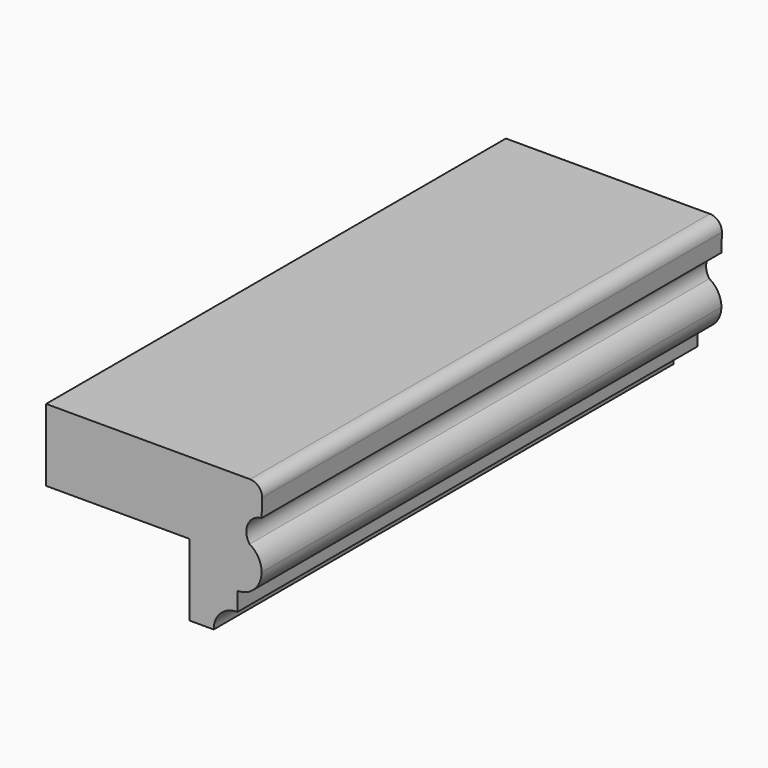
from build123d import *

# Parameters (mm, degrees)
F0_W     = 38.0493849516
F0_H     = 19.1407520324
F1_DEPTH = 152.4


# Not quite as in the source:
# - ends of sketch curves that miss each other by under 0.0002 mm in the source are joined


with BuildPart() as f1:
    # F0 (on Front) → F1 (new body)
    with BuildSketch(Plane.XZ):
        with Locations((-9.5677897334, 9.5703760162)):
            Rectangle(F0_W, F0_H)
        with BuildLine():
            Line((9.4569027424, 19.1407520324), (9.4569027424, 0))
            Line((9.4569027424, 0), (9.4569027424, -19.074914977))
            Line((9.4569027424, -19.074914977), (15.8548746258, -19.074914977))
            ThreePointArc((15.8548746258, -19.074914977), (17.7121304526, -14.6721322023), (22.1616335674, -12.9297724811))
            Line((22.1616335674, -12.9297724811), (22.1616335674, -7.981513619))
            ThreePointArc((22.1616335674, -7.981513619), (26.6843883176, -6.1079115975), (28.5572540015, -1.5848518815))
            ThreePointArc((28.5572540015, -1.5848518815), (27.7056149725, 1.6028958779), (25.3783776729, 3.941914994))
            ThreePointArc((25.3783776729, 3.941914994), (24.8908493588, 8.4306069892), (28.559631396, 11.0623512867))
            Line((28.559631396, 11.0623512867), (28.695607532, 15.8877193117))
            ThreePointArc((28.695607532, 15.8877193117), (27.7740633897, 18.1849926711), (25.4908129573, 19.1407520324))
            Line((25.4908129573, 19.1407520324), (9.4569027424, 19.1407520324))
        make_face()
    extrude(amount=F1_DEPTH)


solid = f1.part
